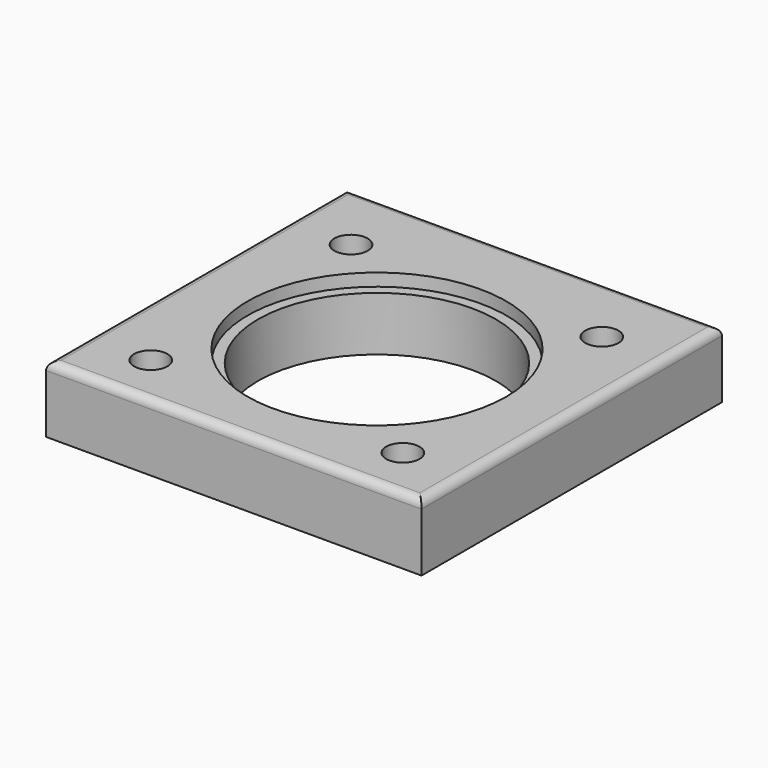
from build123d import *

# Parameters (mm, degrees)
F0_W          = 45
F0_H          = 45
F1_DEPTH      = 8
F2_R          = 14.25
F3_DEPTH      = 69
F3_DEPTH_BACK = 8
F4_W          = 45
F4_H          = 45
F4_R          = 15.5
F5_DEPTH      = 1.5
F6_R          = 1
F7_R          = 2
F8_DEPTH      = 8
F9_DEPTH      = 1.5


# Not quite as in the source:
# - an extrude ends at something that could not be found from the text; its depth is read off the source's solid


with BuildPart() as f1:
    # F0 (on Top) → F1 (new body)
    with BuildSketch(Plane.XY):
        with Locations((-0.144558493, 1.2362819078)):
            Rectangle(F0_W, F0_H)
    extrude(amount=F1_DEPTH)

    # F2 (on face) → F3 (cut, two sides)
    with BuildSketch(Plane.XY.offset(8)) as f3_sk:
        Circle(F2_R)
    extrude(amount=F3_DEPTH, mode=Mode.SUBTRACT)
    extrude(f3_sk.sketch, amount=-F3_DEPTH_BACK, mode=Mode.SUBTRACT)

    # F4 (on face) → F5 (cut)
    with BuildSketch(Plane.XY.offset(8)):
        with Locations((-0.144558493, 1.2362819078)):
            Rectangle(F4_W, F4_H)
        Circle(F4_R, mode=Mode.SUBTRACT)
    extrude(amount=F5_DEPTH, mode=Mode.SUBTRACT)

    # F6
    f6_edges = [f1.edges().sort_by_distance(p)[0] for p in [
        (-0.144558, 23.736282, 8),
        (-22.644558, 1.236282, 8),
        (-0.144558, -21.263718, 8),
        (22.355442, 1.236282, 8),
    ]]
    fillet(f6_edges, radius=F6_R)

    # F7 (on face) → F8 (cut)
    with BuildSketch(Plane.XY.offset(8)):
        with Locations((-15.1081832213, 15)):
            Circle(F7_R)
        with Locations((14.8917229997, 15.0750115548)):
            Circle(F7_R)
        with Locations((15.0417456403, -14.9246133297)):
            Circle(F7_R)
        with Locations((-15.1081832213, -15)):
            Circle(F7_R)
    extrude(amount=-F8_DEPTH, mode=Mode.SUBTRACT)

    # F4 (on face) → F9 (cut)
    with BuildSketch(Plane.XY.offset(8)):
        Circle(F4_R)
    extrude(amount=-F9_DEPTH, mode=Mode.SUBTRACT)


solid = f1.part
